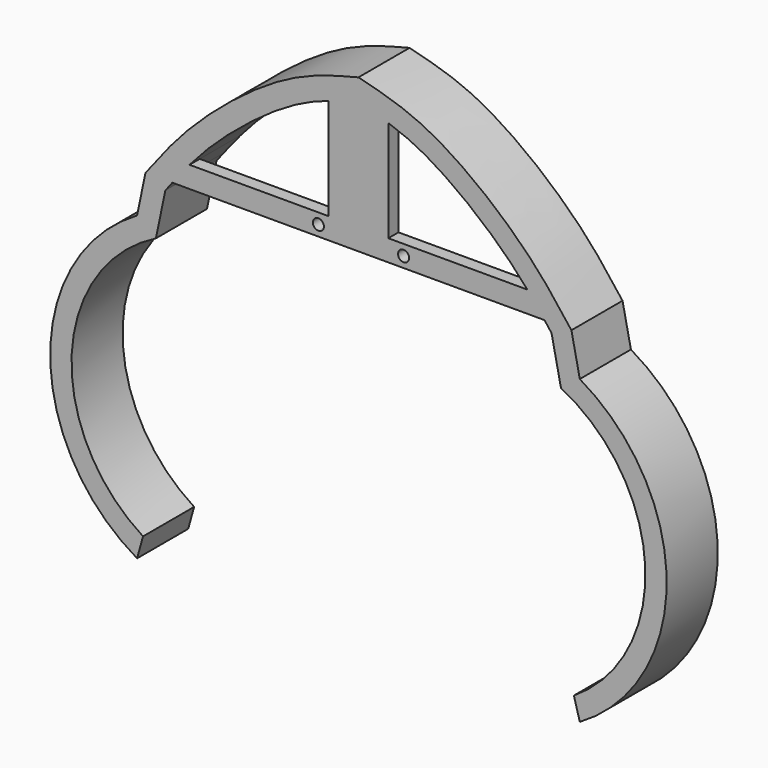
from build123d import *

# Parameters (mm, degrees)
F1_DEPTH = 19.05
F2_R     = 1.651
F3_DEPTH = 25.4
F5_DEPTH = 25.4
F4_W     = 17.78
F4_H     = 30.2702887297
F4_R     = 1.651
F6_DEPTH = 15.24
F9_DEPTH = 25.4


# Not quite as in the source:
# - ends of sketch curves that miss each other by under 0.0002 mm in the source are joined
# - the dataset's text gives a spline's control points without its knots; the knots are read off the source's solid


with BuildPart() as f1:
    # F0 (on Front) → F1 (new body)
    with BuildSketch(Plane.XZ):
        with BuildLine():
            add(Edge.make_bspline(
                [(-63.5, 21.9996418016), (-59.1773038787, 27.7074402987), (-49.5719489383, 40.390596587), (-22.0225745022, 62.1963832768), (-6.7950255866, 66.0154503596), (0, 67.7196418016)],
                knots=[0, 0, 0, 0, 0.3118337223, 0.6929179154, 1, 1, 1, 1], degree=3))
            Line((-63.5, 21.9996418016), (0, 21.9996418016))
            Line((0, 21.9996418016), (0, 67.7196418016))
        make_face()
        with BuildLine():
            Line((0, 67.7196418016), (0, 21.9996418016))
            Line((0, 21.9996418016), (63.5, 21.9996418016))
            add(Edge.make_bspline(
                [(63.5, 21.9996418016), (59.1773038787, 27.7074402987), (49.5719489383, 40.390596587), (22.0225745022, 62.1963832768), (6.7950255866, 66.0154503596), (0, 67.7196418016)],
                knots=[0, 0, 0, 0, 0.3118337223, 0.6929179154, 1, 1, 1, 1], degree=3))
        make_face()
        Polygon((0, 21.9996418016), (-63.5, 21.9996418016), (-66, 9.9996418016), (66, 9.9996418016), (63.5, 21.9996418016), align=None)
        with BuildLine():
            Line((-66, -80.0003581984), (-66, 9.9996418016))
            ThreePointArc((-66, 9.9996418016), (-91.9025448723, -35.0003581984), (-66, -80.0003581984))
        make_face()
        with BuildLine():
            Line((66, 9.9996418016), (-66, 9.9996418016))
            Line((-66, 9.9996418016), (-66, -80.0003581984))
            Line((-66, -80.0003581984), (66, -80.0003581984))
            ThreePointArc((66, -80.0003581984), (91.9025448723, -35.0003581984), (66, 9.9996418016))
        make_face()
    extrude(amount=F1_DEPTH)

    # F2 (on face) → F3 (cut)
    with BuildSketch(Plane.XZ.offset(19.05)):
        with Locations((-11.9451396167, 25.2144485712)):
            Circle(F2_R)
        with Locations((13.4548603833, 25.2144485712)):
            Circle(F2_R)
    extrude(amount=-F3_DEPTH, mode=Mode.SUBTRACT)

    # F4 (on face) → F5 (cut)
    with BuildSketch(Plane(origin=(0, 0, 0), x_dir=(-1, 0, 0), z_dir=(0, 1, 0))):
        with BuildLine():
            add(Edge.make_bspline(
                [(8.8899999224, 58.6597370674), (9.4174668563, 58.4844301364), (10.6027253629, 58.0760317288), (12.4528066572, 57.3811446045), (14.1186878127, 56.6903543188), (15.465576075, 56.087988482), (16.4840604895, 55.6094842125), (17.3407970771, 55.1868451521), (18.0314759833, 54.8334983404), (18.7262436543, 54.4694480455), (19.6075281463, 53.9915801734), (21.0395239737, 53.18172973), (22.8650854165, 52.0886083872), (25.0932846475, 50.6624104213), (27.3413431054, 49.1365546816), (29.5924177005, 47.5259285779), (31.8303604349, 45.8454314349), (34.0394820405, 44.1099993889), (36.2044115804, 42.3346300454), (38.3099635298, 40.5344399502), (40.341056744, 38.7247117719), (41.958938324, 37.2216929551), (43.20091501, 36.0302372367), (44.1040049121, 35.144495274), (44.9779614296, 34.2674991508), (46.1087390929, 33.1068486062), (47.4606258693, 31.6717601272), (48.9653058522, 30.0052513316), (49.9124061795, 28.9152673121), (50.3616732575, 28.3894485712)],
                knots=[0.1624327167, 0.1624327167, 0.1624327167, 0.1624327167, 0.1875, 0.21875, 0.25, 0.265625, 0.28125, 0.296875, 0.3046875, 0.3125, 0.328125, 0.34375, 0.375, 0.40625, 0.4375, 0.46875, 0.5, 0.53125, 0.5625, 0.59375, 0.625, 0.65625, 0.671875, 0.6875, 0.703125, 0.71875, 0.75, 0.78125, 0.8105240349, 0.8105240349, 0.8105240349, 0.8105240349], degree=3))
            Line((8.8899999224, 58.6597370674), (8.89, 28.3894485712))
            Line((8.89, 28.3894485712), (50.3616732575, 28.3894485712))
        make_face()
        with BuildLine():
            Line((-8.89, 28.3894485712), (-8.89, 58.6597373009))
            add(Edge.make_bspline(
                [(-50.3616732575, 28.3894485712), (-49.9124061795, 28.9152673121), (-48.9653058522, 30.0052513316), (-47.4606258693, 31.6717601272), (-46.1087390929, 33.1068486062), (-44.9779614296, 34.2674991508), (-44.1040049121, 35.144495274), (-43.20091501, 36.0302372367), (-41.958938324, 37.2216929551), (-40.341056744, 38.7247117719), (-38.3099635298, 40.5344399502), (-36.2044115804, 42.3346300454), (-34.0394820405, 44.1099993889), (-31.8303604349, 45.8454314349), (-29.5924177005, 47.5259285779), (-27.3413431054, 49.1365546816), (-25.0932846475, 50.6624104213), (-22.8650854165, 52.0886083872), (-21.0395239737, 53.18172973), (-19.6075281463, 53.9915801734), (-18.7262436543, 54.4694480455), (-18.0314759833, 54.8334983404), (-17.3407970771, 55.1868451521), (-16.4840604895, 55.6094842125), (-15.465576075, 56.087988482), (-14.1186878127, 56.6903543188), (-12.4528066572, 57.3811446045), (-10.6027253629, 58.0760317288), (-9.4174668563, 58.4844301364), (-8.89, 58.6597373009)],
                knots=[0.1894759651, 0.1894759651, 0.1894759651, 0.1894759651, 0.21875, 0.25, 0.28125, 0.296875, 0.3125, 0.328125, 0.34375, 0.375, 0.40625, 0.4375, 0.46875, 0.5, 0.53125, 0.5625, 0.59375, 0.625, 0.65625, 0.671875, 0.6875, 0.6953125, 0.703125, 0.71875, 0.734375, 0.75, 0.78125, 0.8125, 0.8375672833, 0.8375672833, 0.8375672833, 0.8375672833], degree=3))
            Line((-50.3616732575, 28.3894485712), (-8.89, 28.3894485712))
        make_face()
        with BuildLine():
            Line((55.4861742022, 22.0394485712), (-55.4861742022, 22.0394485712))
            add(Edge.make_bspline(
                [(-57.5751450411, 19.3044778842), (-56.9999128128, 20.0628115549), (-56.3059239214, 20.9747923821), (-55.6075086455, 21.8821649038), (-55.4861742022, 22.0394485712)],
                knots=[0.0208024, 0.0208024, 0.0208024, 0.0208024, 0.0625, 0.071251624, 0.071251624, 0.071251624, 0.071251624], degree=3))
            Line((-57.5751450411, 19.3044778842), (-60.3840423883, 5.8218056306))
            ThreePointArc((-60.3840423883, 5.8218056306), (-85.4991451839, -32.7920053667), (-64.229688396, -73.6503581984))
            Line((-64.229688396, -73.6503581984), (64.229688396, -73.6503581984))
            ThreePointArc((64.229688396, -73.6503581984), (85.4991451839, -32.7920053667), (60.3840423883, 5.8218056306))
            Line((60.3840423883, 5.8218056306), (57.57515134, 19.3044826623))
            add(Edge.make_bspline(
                [(55.4861742022, 22.0394485712), (55.6075086455, 21.8821649038), (56.3059239214, 20.9747923821), (56.9999128128, 20.0628115549), (57.57515134, 19.3044826623)],
                knots=[0.928748376, 0.928748376, 0.928748376, 0.928748376, 0.9375, 0.9791976, 0.9791976, 0.9791976, 0.9791976], degree=3))
        make_face()
    extrude(amount=-F5_DEPTH, mode=Mode.SUBTRACT)

    # F4 (on face) → F6 (cut)
    with BuildSketch(Plane(origin=(0, 0, 0), x_dir=(-1, 0, 0), z_dir=(0, 1, 0))):
        with Locations((0, 43.5245929361)):
            Rectangle(F4_W, F4_H)
        with BuildLine():
            Line((-8.89, 28.3894485712), (-50.3616732575, 28.3894485712))
            add(Edge.make_bspline(
                [(-55.4861742022, 22.0394485712), (-54.7409948713, 23.0054112021), (-53.5519640772, 24.5257325033), (-51.867677946, 26.6026767314), (-50.9012395069, 27.7572590438), (-50.3919982895, 28.3539563864), (-50.3616732575, 28.3894485712)],
                knots=[0.071251624, 0.071251624, 0.071251624, 0.071251624, 0.125, 0.15625, 0.1875, 0.1894759651, 0.1894759651, 0.1894759651, 0.1894759651], degree=3))
            Line((-55.4861742022, 22.0394485712), (55.4861742022, 22.0394485712))
            add(Edge.make_bspline(
                [(50.3616732575, 28.3894485712), (50.3919982895, 28.3539563864), (50.9012395069, 27.7572590438), (51.867677946, 26.6026767314), (53.5519640772, 24.5257325033), (54.7409948713, 23.0054112021), (55.4861742022, 22.0394485712)],
                knots=[0.8105240349, 0.8105240349, 0.8105240349, 0.8105240349, 0.8125, 0.84375, 0.875, 0.928748376, 0.928748376, 0.928748376, 0.928748376], degree=3))
            Line((50.3616732575, 28.3894485712), (8.89, 28.3894485712))
            Line((8.89, 28.3894485712), (-8.89, 28.3894485712))
        make_face()
        with Locations((-13.4548603833, 25.2144485712)):
            Circle(F4_R, mode=Mode.SUBTRACT)
        with Locations((11.9451396167, 25.2144485712)):
            Circle(F4_R, mode=Mode.SUBTRACT)
        with Locations((11.9451396167, 25.2144485712)):
            Circle(F4_R)
    extrude(amount=-F6_DEPTH, mode=Mode.SUBTRACT)

    # F8 (on face) → F9 (cut)
    with BuildSketch(Plane.XZ.offset(19.05)):
        with BuildLine():
            ThreePointArc((-60.3840423883, 5.8218056306), (-85.4991451839, -32.7920053667), (-64.229688396, -73.6503581984))
            Line((-64.229688396, -73.6503581984), (64.229688396, -73.6503581984))
            ThreePointArc((64.229688396, -73.6503581984), (85.4991451839, -32.7920053667), (60.3840423883, 5.8218056306))
            Line((60.3840423883, 5.8218056306), (57.5751450411, 19.3044778842))
            add(Edge.make_bspline(
                [(55.4861742022, 22.0394485712), (55.7717659543, 21.6692410939), (56.0565718474, 21.29842749), (56.340705921, 20.9270989722), (56.6243014781, 20.5553596846), (57.04117319, 20.0076596246), (57.1747707101, 19.8319436665), (57.3082896056, 19.6561679183), (57.4417432663, 19.480342609), (57.5751450411, 19.3044778842)],
                knots=[0, 0, 0, 0, 0, 0, 0.6793028355, 0.6793028355, 0.6793028355, 0.6793028355, 1, 1, 1, 1, 1, 1], degree=5))
            Line((55.4861742022, 22.0394485712), (-55.4861742022, 22.0394485712))
            add(Edge.make_bspline(
                [(-57.57515134, 19.3044826623), (-57.2164741279, 19.7773218067), (-56.8574238872, 20.2498772648), (-56.497740911, 20.7219524543), (-56.1371602712, 21.1933427545), (-55.7176373022, 21.739014281), (-55.6598180579, 21.8141586931), (-55.6019684458, 21.889279733), (-55.5440874851, 21.964376619), (-55.4861742022, 22.0394485712)],
                knots=[0, 0, 0, 0, 0, 0, 0.8622486286, 0.8622486286, 0.8622486286, 0.8622486286, 1, 1, 1, 1, 1, 1], degree=5))
            Line((-57.57515134, 19.3044826623), (-60.3840423883, 5.8218056306))
        make_face()
        Polygon((64.229688396, -73.6503581984), (-64.229688396, -73.6503581984), (-66, -80.0003581984), (66, -80.0003581984), align=None)
    extrude(amount=-F9_DEPTH, mode=Mode.SUBTRACT)


solid = f1.part
